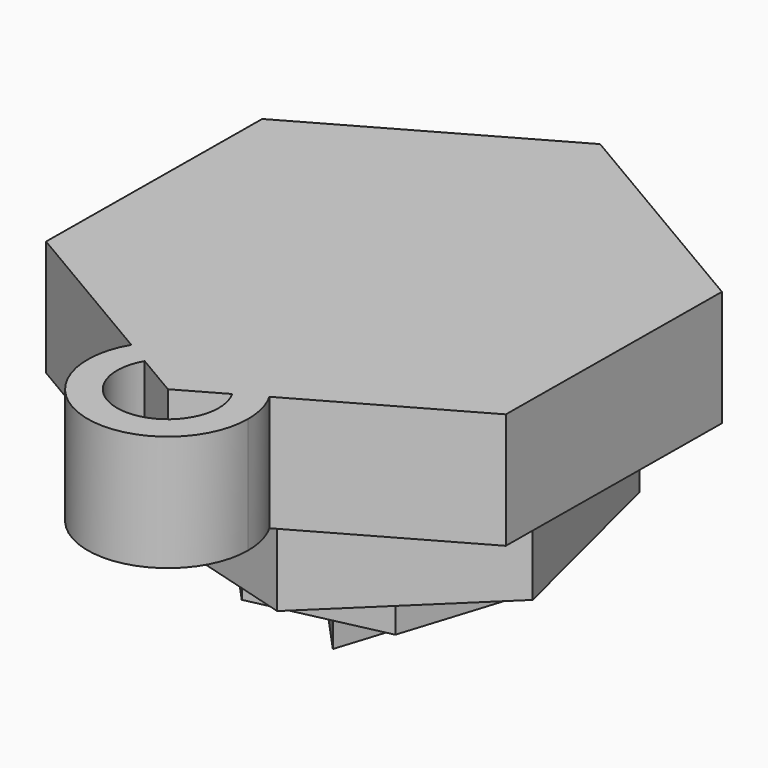
from build123d import *

# Parameters (mm, degrees)
F1_DEPTH     = 6.35
F3_DEPTH     = 5.08
F5_DEPTH     = 2.54
F7_DEPTH     = 2.032
F8_TEXT_SIZE = 5.2514709927
F9_DEPTH     = 2.54
F11_DEPTH    = 6.35


# Not quite as in the source:
# - Text() gives the source's letters only with a copy of the font that has no kerning and outlines rounded to 1/6400 em; it was checked with that copy


with BuildPart() as f1:
    # F0 (on Top) → F1 (new body)
    with BuildSketch(Plane.XY):
        Polygon((-0.1266545273, -14.6641498889), (12.636199065, -7.4417609826), (12.7628535924, 7.2223889063), (0.1266545273, 14.6641498889), (-12.636199065, 7.4417609826), (-12.7628535924, -7.2223889063), align=None)
    extrude(amount=-F1_DEPTH)

    # F10 (on face) → F11 (join)
    with BuildSketch(Plane(origin=(0, 0, -6.35), x_dir=(1, 0, 0), z_dir=(0, 0, -1))):
        with BuildLine():
            ThreePointArc((3.7087809269, 12.4937100045), (4.1350363915, 13.5419355922), (4.2803143194, 14.6641498889))
            ThreePointArc((4.2803143194, 14.6641498889), (-1.2856338974, 18.915989636), (-3.9240283317, 12.4277852931))
            Line((-3.9240283317, 12.4277852931), (-2.5314504586, 13.2479078338))
            ThreePointArc((-2.5314504586, 13.2479078338), (-0.8606114716, 17.3567494198), (2.6641849575, 14.6641498889))
            ThreePointArc((2.6641849575, 14.6641498889), (2.5721835408, 13.9534754824), (2.302245036, 13.289656549))
            Line((2.302245036, 13.289656549), (3.7087809269, 12.4937100045))
        make_face()
    extrude(amount=-F11_DEPTH)


with BuildPart() as f3:
    # F2 (on face) → F3 (new body)
    with BuildSketch(Plane(origin=(0, 0, -6.35), x_dir=(1, 0, 0), z_dir=(0, 0, -1))):
        Polygon((-2.6739730165, -10.6685223113), (7.9022248342, -7.649989717), (10.5761978507, 3.0185325944), (2.6739730165, 10.6685223113), (-7.9022248342, 7.649989717), (-10.5761978507, -3.0185325944), align=None)
    extrude(amount=F3_DEPTH)

    # F4 (on face) → F5 (join)
    with BuildSketch(Plane(origin=(0, 0, -11.43), x_dir=(1, 0, 0), z_dir=(0, 0, -1))):
        Polygon((2.2122408485, -6.9906597515), (7.1602093583, -1.5794731017), (4.9479685098, 5.4111866498), (-2.2122408485, 6.9906597515), (-7.1602093583, 1.5794731017), (-4.9479685098, -5.4111866498), align=None)
    extrude(amount=F5_DEPTH)


with BuildPart() as f7:
    # F6 (on face) → F7 (new body)
    with BuildSketch(Plane(origin=(0, 0, -13.97), x_dir=(1, 0, 0), z_dir=(0, 0, -1))):
        Polygon((1.2491711648, 5.0719101076), (-5.5287618227, -2.3405583474), (4.2795906579, -4.5041862722), align=None)
    extrude(amount=F7_DEPTH)

    # F8 (on face) → F9 (cut)
    with BuildSketch(Plane(origin=(0, 0, -16.002), x_dir=(1, 0, 0), z_dir=(0, 0, -1))):
        with Locations((-2.1397953289, -2.4153832346)):
            Text('B', F8_TEXT_SIZE, font='Open Sans', text_align=(TextAlign.LEFT, TextAlign.BOTTOM))
    extrude(amount=-F9_DEPTH, mode=Mode.SUBTRACT)


solid = Compound([f1.part, f3.part, f7.part])
